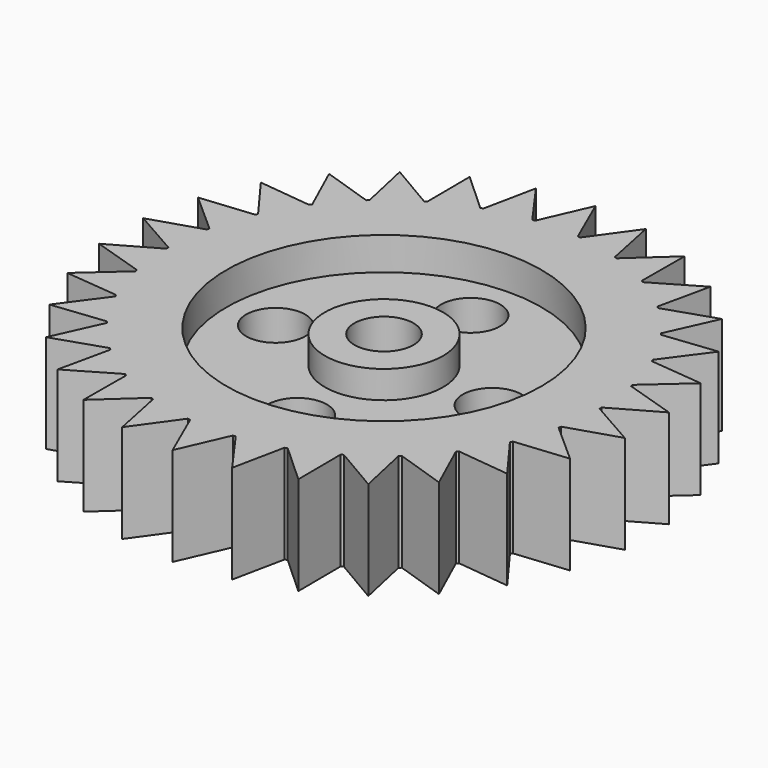
from build123d import *

# Parameters (mm, degrees)
F0_R             = 13.97
F1_DEPTH         = 3.175
F2_R             = 10.16
F3_DEPTH         = 2.1166666667
F4_R             = 10.16
F5_DEPTH         = 2.1166666667
F6_R             = 1.905
F7_DEPTH         = 2.54
F7_COPIES_COUNT  = 4
F8_R             = 3.81
F9_DEPTH         = 1.778
F10_R            = 3.81
F11_DEPTH        = 1.778
F13_DEPTH        = 6.35
F13_COPIES_COUNT = 30
F14_R            = 1.905
F15_DEPTH        = 5.6726666667


# Not quite as in the source:
# - a pattern or mirror of a feature is missing from the dataset's text; its kind, count and spacing are read off the source's solid


with BuildPart() as f1:
    # F0 (on Top) → F1 (new body, symmetric)
    with BuildSketch(Plane.XY):
        Circle(F0_R)
    extrude(amount=F1_DEPTH, both=True)

    # F2 (on face) → F3 (cut)
    with BuildSketch(Plane.XY.offset(3.175)):
        Circle(F2_R)
    extrude(amount=-F3_DEPTH, mode=Mode.SUBTRACT)

    # F4 (on face) → F5 (cut)
    with BuildSketch(Plane(origin=(0, 0, -3.175), x_dir=(1, 0, 0), z_dir=(0, 0, -1))):
        Circle(F4_R)
    extrude(amount=-F5_DEPTH, mode=Mode.SUBTRACT)

    # F6 (on face) → F7 (cut)
    with BuildSketch(Plane.XY.offset(1.0583333333)):
        with Locations((0, 6.985)):
            Circle(F6_R)
    f7 = extrude(amount=-F7_DEPTH, mode=Mode.SUBTRACT)

    # F7_copies: F7 ×4 about axis
    f7_copies_axis = Axis((0, 0, 0), (0, 0, 1))
    for i in range(1, F7_COPIES_COUNT):
        add(f7.rotate(f7_copies_axis, i * 360 / F7_COPIES_COUNT), mode=Mode.SUBTRACT)

    # F8 (on face) → F9 (join)
    with BuildSketch(Plane.XY.offset(1.0583333333)):
        Circle(F8_R)
    extrude(amount=F9_DEPTH)

    # F10 (on face) → F11 (join)
    with BuildSketch(Plane(origin=(0, 0, -1.0583333333), x_dir=(1, 0, 0), z_dir=(0, 0, -1))):
        Circle(F10_R)
    extrude(amount=F11_DEPTH)

    # F12 (on face) → F13 (join, through all)
    with BuildSketch(Plane.XY.offset(3.175)):
        Polygon((0, 17.0471984893), (-1.3763362913, 13.9020357651), (1.3763362913, 13.9020357651), align=None)
    f13 = extrude(amount=-F13_DEPTH)

    # F13_copies: F13 ×30 about axis
    f13_copies_axis = Axis((0, 0, 0), (0, 0, 1))
    for i in range(1, F13_COPIES_COUNT):
        add(f13.rotate(f13_copies_axis, i * 360 / F13_COPIES_COUNT))

    # F14 (on face) → F15 (cut, through all)
    with BuildSketch(Plane.XY.offset(2.8363333333)):
        Circle(F14_R)
    extrude(amount=-F15_DEPTH, mode=Mode.SUBTRACT)


solid = f1.part
